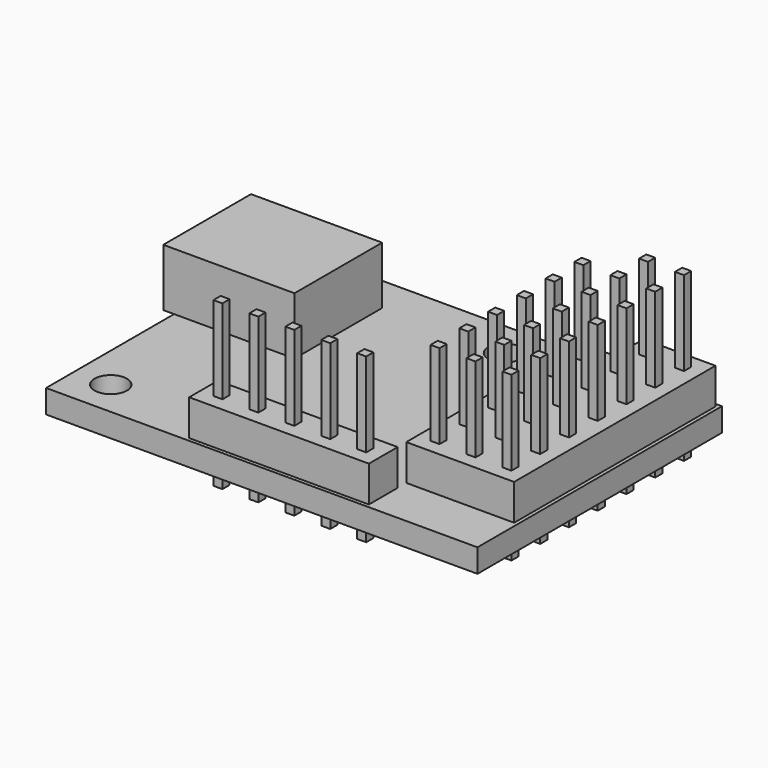
from build123d import *

# Parameters (mm, degrees)
F0_W          = 30.48
F0_H          = 21.59
F0_R          = 1.143
F1_DEPTH      = 1.651
F3_DEPTH      = 2.54
F2_W          = 12.7
F2_H          = 2.54
F4_W          = 0.635
F4_H          = 0.635
F5_DEPTH      = 5.969
F5_DEPTH_BACK = 5.588
F6_DEPTH      = 5.969
F6_DEPTH_BACK = 5.588
F7_W          = 9.271
F7_H          = 7.747
F8_DEPTH      = 4.064


with BuildPart() as f1:
    # F0 (on Top) → F1 (new body)
    with BuildSketch(Plane.XY):
        with Locations((15.24, 10.795)):
            Rectangle(F0_W, F0_H)
        with Locations((2.54, 2.54)):
            Circle(F0_R, mode=Mode.SUBTRACT)
        with Locations((17.145, 19.05)):
            Circle(F0_R, mode=Mode.SUBTRACT)
    extrude(amount=F1_DEPTH)


with BuildPart() as f3:
    # F2 (on face) → F3 (new body)
    with BuildSketch(Plane.XY.offset(1.651)):
        Polygon((30.226, 3.556), (30.226, 21.336), (25.146, 21.336), (25.146, 18.796), (22.606, 18.796), (22.606, 3.556), align=None)
    extrude(amount=F3_DEPTH)

    # F4 (on face) → F6 (join, two sides)
    with BuildSketch(Plane.XY.offset(4.191)) as f6_sk:
        with Locations((23.876, 9.906)):
            Rectangle(F4_W, F4_H)
        with Locations((28.956, 7.366)):
            Rectangle(F4_W, F4_H)
        with Locations((26.416, 14.986)):
            Rectangle(F4_W, F4_H)
        with Locations((26.416, 9.906)):
            Rectangle(F4_W, F4_H)
        with Locations((26.416, 17.526)):
            Rectangle(F4_W, F4_H)
        with Locations((26.416, 12.446)):
            Rectangle(F4_W, F4_H)
        with Locations((26.416, 4.826)):
            Rectangle(F4_W, F4_H)
        with Locations((26.416, 7.366)):
            Rectangle(F4_W, F4_H)
        with Locations((28.956, 17.526)):
            Rectangle(F4_W, F4_H)
        with Locations((23.876, 17.526)):
            Rectangle(F4_W, F4_H)
        with Locations((23.876, 7.366)):
            Rectangle(F4_W, F4_H)
        with Locations((23.876, 4.826)):
            Rectangle(F4_W, F4_H)
        with Locations((28.956, 12.446)):
            Rectangle(F4_W, F4_H)
        with Locations((23.876, 14.986)):
            Rectangle(F4_W, F4_H)
        with Locations((23.876, 12.446)):
            Rectangle(F4_W, F4_H)
        with Locations((28.956, 9.906)):
            Rectangle(F4_W, F4_H)
        with Locations((28.956, 14.986)):
            Rectangle(F4_W, F4_H)
        with Locations((28.956, 4.826)):
            Rectangle(F4_W, F4_H)
        with Locations((28.956, 20.066)):
            Rectangle(F4_W, F4_H)
        with Locations((26.416, 20.066)):
            Rectangle(F4_W, F4_H)
    extrude(amount=F6_DEPTH)
    extrude(f6_sk.sketch, amount=-F6_DEPTH_BACK)


with BuildPart() as f3b:
    # F2 (on face) → F3, piece 2 (new body)
    with BuildSketch(Plane.XY.offset(1.651)):
        with Locations((16.256, 1.524)):
            Rectangle(F2_W, F2_H)
    extrude(amount=F3_DEPTH)

    # F4 (on face) → F5 (join, two sides)
    with BuildSketch(Plane.XY.offset(4.191)) as f5_sk:
        with Locations((21.336, 1.524)):
            Rectangle(F4_W, F4_H)
        with Locations((18.796, 1.524)):
            Rectangle(F4_W, F4_H)
        with Locations((16.256, 1.524)):
            Rectangle(F4_W, F4_H)
        with Locations((13.716, 1.524)):
            Rectangle(F4_W, F4_H)
        with Locations((11.176, 1.524)):
            Rectangle(F4_W, F4_H)
    extrude(amount=F5_DEPTH)
    extrude(f5_sk.sketch, amount=-F5_DEPTH_BACK)


with BuildPart() as f8:
    # F7 (on face) → F8 (new body)
    with BuildSketch(Plane.XY.offset(1.651)):
        with Locations((3.8735, 15.1765)):
            Rectangle(F7_W, F7_H)
    extrude(amount=F8_DEPTH)


solid = Compound([f1.part, f3.part, f3b.part, f8.part])
